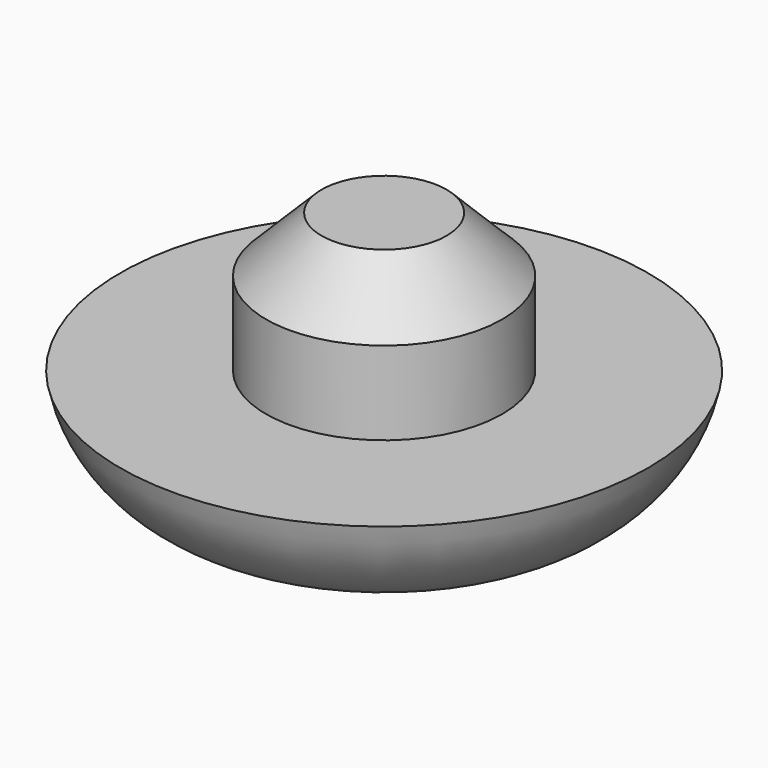
from build123d import *

# Parameters (mm, degrees)
F0_R     = 9.5
F1_DEPTH = 4
F2_R     = 4.25
F3_DEPTH = 5
F5_SIZE  = 2
F6_DEPTH = 1


# Not quite as in the source:
# - a fillet or chamfer that OpenCascade refuses, or shapes differently, is made with other operations: its cross-section is extruded or revolved along the edge and cut away or added


with BuildPart() as f1:
    # F0 (on Top) → F1 (new body)
    with BuildSketch(Plane.XY):
        Circle(F0_R)
    extrude(amount=F1_DEPTH)

    # F2 (on face) → F3 (join)
    with BuildSketch(Plane.XY.offset(4)):
        Circle(F2_R)
    extrude(amount=F3_DEPTH)

    # F4: fillet of radius 5 on 1 edges, made by hand

    # F4_s1 → F4_t2 (revolve, cut)
    with BuildSketch(Plane.XZ):
        with BuildLine():
            ThreePointArc((9.5, 4), (7.7632981746, 1.1270166538), (4.6010205144, 0))
            Line((4.6010205144, 0), (9.5, 0))
            Line((9.5, 0), (9.5, 4))
        make_face()
    revolve(axis=Axis((0, 0, 0), (0, 0, 1)), mode=Mode.SUBTRACT)

    # F5
    f5_edges = [f1.edges().sort_by_distance(p)[0] for p in [
        (-4.25, 0, 9),
    ]]
    chamfer(f5_edges, length=F5_SIZE)

    # F6 (cut): a face of the model
    f6_faces = [f1.faces().sort_by_distance(p)[0] for p in [
        (0, 0, 0),
    ]]
    extrude(f6_faces, amount=-F6_DEPTH, mode=Mode.SUBTRACT)

    # F7: fillet of radius 2 on 1 edges, made by hand

    # F7_s1 → F7_t2 (revolve, cut)
    with BuildSketch(Plane.XZ):
        with BuildLine():
            ThreePointArc((7.0216351058, 0.625), (5.7472030514, 0.3985764624), (4.6010205144, 1))
            Line((4.6010205144, 1), (4.6010205144, 0))
            ThreePointArc((4.6010205144, 0), (5.8510205144, 0.1587708172), (7.0216351058, 0.625))
        make_face()
    revolve(axis=Axis((0, 0, 0), (0, 0, 1)), mode=Mode.SUBTRACT)


solid = f1.part
